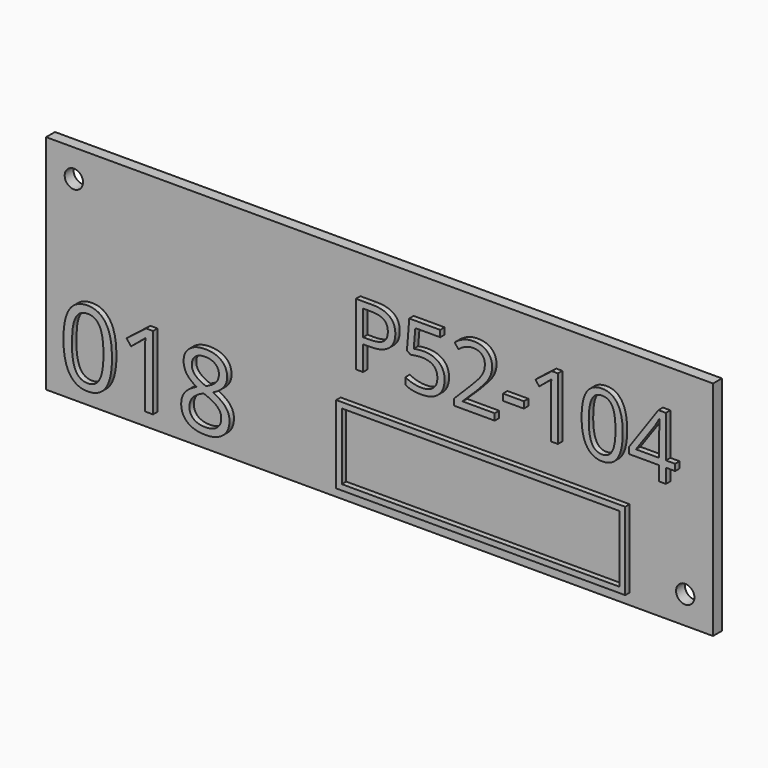
from build123d import *

# Parameters (mm, degrees)
F0_W         = 120
F0_H         = 40
F1_DEPTH     = 2
F3_D         = 3.3
F4_TEXT_SIZE = 15.6773087287
F5_DEPTH     = 1
F6_TEXT_SIZE = 18.5155049272
F7_DEPTH     = 1
F8_W         = 52
F8_H         = 14
F8_W_2       = 49.99999962
F8_H_2       = 11.99999962
F9_DEPTH     = 1


# Not quite as in the source:
# - Text() gives the source's letters only with a copy of the font that has no kerning and outlines rounded to 1/6400 em; it was checked with that copy


with BuildPart() as f1:
    # F0 (on Front) → F1 (new body)
    with BuildSketch(Plane.XZ):
        Rectangle(F0_W, F0_H)
    extrude(amount=F1_DEPTH)

    # F3 (through all)
    with Locations(Plane.XZ.offset(2)):
        with Locations((-55, 15), (55, -15)):
            Hole(F3_D / 2)

    # F4 (on face) → F5 (join)
    with BuildSketch(Plane.XZ.offset(2)):
        with Locations((-5, 2)):
            Text('P52-104', F4_TEXT_SIZE, font='Open Sans', text_align=(TextAlign.LEFT, TextAlign.BOTTOM))
    extrude(amount=F5_DEPTH)

    # F6 (on face) → F7 (join)
    with BuildSketch(Plane.XZ.offset(2)):
        with Locations((-57, -17)):
            Text('018', F6_TEXT_SIZE, font='Open Sans', text_align=(TextAlign.LEFT, TextAlign.BOTTOM))
    extrude(amount=F7_DEPTH)

    # F8 (on face) → F9 (join)
    with BuildSketch(Plane.XZ.offset(2)):
        with Locations((19, -11)):
            Rectangle(F8_W, F8_H)
        with Locations((19, -11)):
            Rectangle(F8_W_2, F8_H_2, mode=Mode.SUBTRACT)
    extrude(amount=F9_DEPTH)


solid = f1.part
